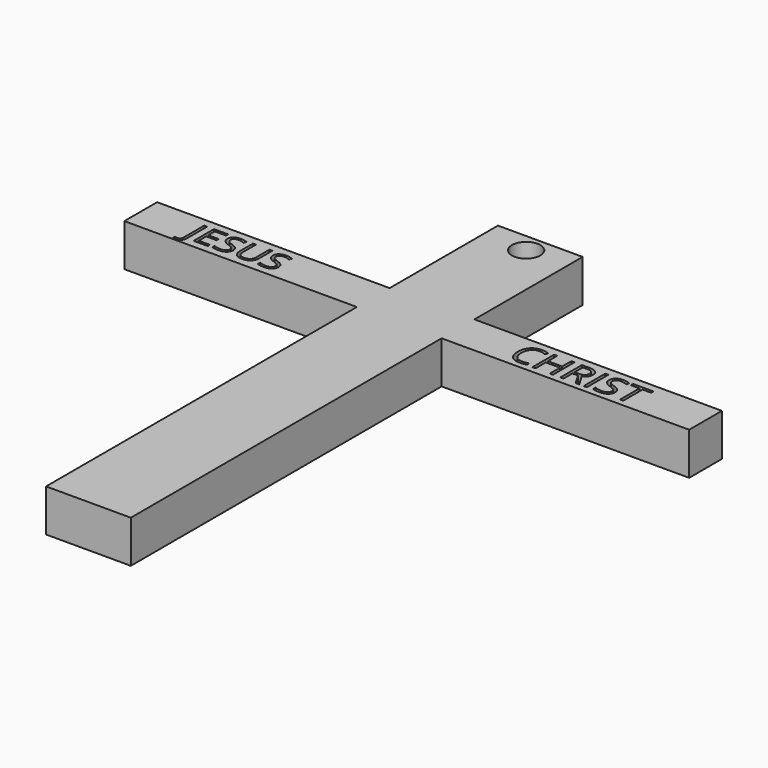
from build123d import *

# Parameters (mm, degrees)
F0_W         = 7.62
F0_H         = 50.8
F1_DEPTH     = 3.81
F2_W         = 50.8
F2_H         = 3.683
F3_DEPTH     = 3.81
F4_R         = 1.2739606307
F5_DEPTH     = 3.811
F6_TEXT_SIZE = 3.1978415791
F7_DEPTH     = 2.54
F8_TEXT_SIZE = 3.3977066374
F9_DEPTH     = 2.54


# Not quite as in the source:
# - Text() gives the source's letters only with a copy of the font that has no kerning and outlines rounded to 1/6400 em; it was checked with that copy


with BuildPart() as f1:
    # F0 (on Top) → F1 (new body)
    with BuildSketch(Plane.XY):
        with Locations((-0.0819488434, -13.2271464258)):
            Rectangle(F0_W, F0_H)
    extrude(amount=F1_DEPTH)

    # F2 (on Top) → F3 (join)
    with BuildSketch(Plane.XY):
        with Locations((0.5905532002, -1.8415)):
            Rectangle(F2_W, F2_H)
    extrude(amount=F3_DEPTH)

    # F4 (on Top) → F5 (cut, through all)
    with BuildSketch(Plane.XY):
        with Locations((0, 10.4799941182)):
            Circle(F4_R)
    extrude(amount=F5_DEPTH, mode=Mode.SUBTRACT)

    # F6 (on face) → F7 (cut)
    with BuildSketch(Plane.XY.offset(3.81)):
        with Locations((-20.297197625, -2.9892295133)):
            Text('JESUS', F6_TEXT_SIZE, font='Open Sans', text_align=(TextAlign.LEFT, TextAlign.BOTTOM))
    extrude(amount=-F7_DEPTH, mode=Mode.SUBTRACT)

    # F8 (on face) → F9 (cut)
    with BuildSketch(Plane.XY.offset(3.81)):
        with Locations((8.9748445898, -3.1278457027)):
            Text('CHRIST', F8_TEXT_SIZE, font='Open Sans', text_align=(TextAlign.LEFT, TextAlign.BOTTOM))
    extrude(amount=-F9_DEPTH, mode=Mode.SUBTRACT)


solid = f1.part
